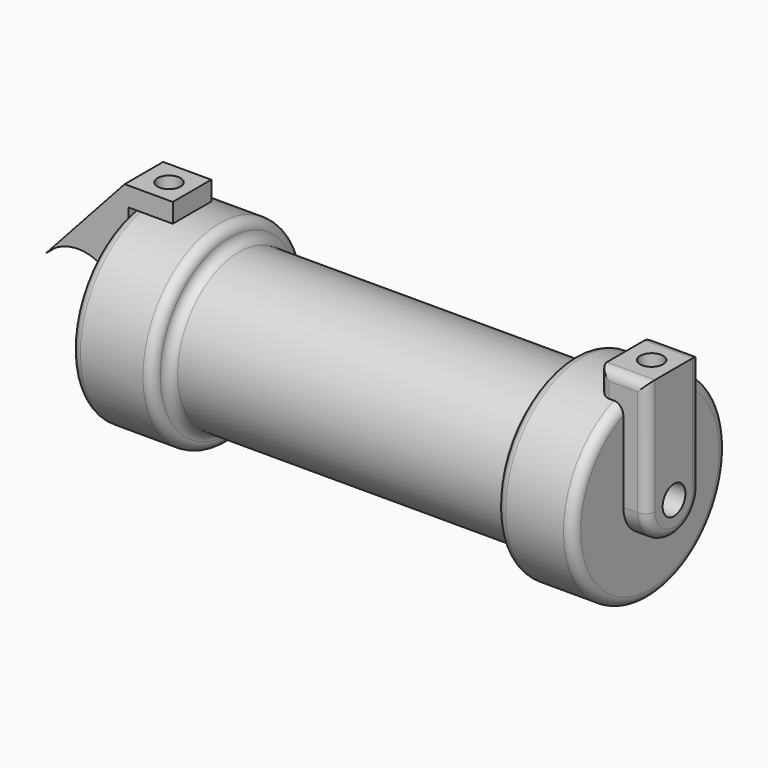
from build123d import *

# Parameters (mm, degrees)
F0_W     = 5.842
F0_H     = 12.7
F2_DEPTH = 3.175
F3_DEPTH = 0.635
F5_D     = 3.048
F5_DEPTH = 17.78
F5_TIP   = 0.9157115834
F6_R     = 1.8819905546
F7_DEPTH = 3.175
F9_D     = 3.048
F9_DEPTH = 10.414
F9_TIP   = 0.9157115834
F10_R    = 1.27
F11_R    = 1.26999


# Not quite as in the source:
# - two fillets or chamfers of one size are made in one step
# - a fillet or chamfer is up to 0.001 mm smaller than in the source, because OpenCascade refuses the exact size
# - a feature of the source that left no trace in its solid (it failed there, or was rolled back) is left out


with BuildPart() as f1:
    # F0 (on Front) → F1 (revolve)
    with BuildSketch(Plane.XZ):
        Polygon((5.842, 12.7), (5.842, 0), (66.294, 0), (66.294, 12.7), (56.134, 12.7), (56.134, 10.16), (10.16, 10.16), (10.16, 12.7), align=None)
        with Locations((2.921, 6.35)):
            Rectangle(F0_W, F0_H)
    revolve(axis=Axis((33.147, 0, 0), (-1, 0, 0)))

    # F3 (add, symmetric): a face of the model
    f3_faces = [f1.faces().sort_by_distance(p)[0] for p in [
        (10.16, 0, -10.5192102448),
    ]]
    extrude(f3_faces, amount=F3_DEPTH, both=True)

    # F6 (on face) → F7 (join, symmetric)
    with BuildSketch(Plane.YZ.offset(66.294)):
        with BuildLine():
            Line((-4.4024969223, 15.2352917939), (-4.4024969223, 11.9125153032))
            ThreePointArc((-4.4024969223, 11.9125153032), (-0.0272881349, 12.6999706833), (4.3512642127, 11.9313243084))
            Line((4.3512642127, 11.9313243084), (4.3512642127, 15.2352917939))
            Line((4.3512642127, 15.2352917939), (-0.0256163548, 15.2352917939))
            Line((-0.0256163548, 15.2352917939), (-4.4024969223, 15.2352917939))
        make_face()
        with BuildLine():
            Line((-4.4024969223, 11.9125153032), (-4.4024969223, 0.0887250123))
            ThreePointArc((-4.4024969223, 0.0887250123), (-0.2945224047, 4.3935302243), (4.3512642127, 0.6755375863))
            Line((4.3512642127, 0.6755375863), (4.3512642127, 11.9313243084))
            ThreePointArc((4.3512642127, 11.9313243084), (-0.0272881349, 12.6999706833), (-4.4024969223, 11.9125153032))
        make_face()
        with BuildLine():
            Line((-4.4024969223, 0.0887250123), (-4.4024969223, -0.0887250123))
            ThreePointArc((-4.4024969223, -0.0887250123), (0.0443647579, -4.403167388), (4.4033908842, 0))
            ThreePointArc((4.4033908842, 0), (4.3903398756, 0.3387728665), (4.3512642127, 0.6755375863))
            ThreePointArc((4.3512642127, 0.6755375863), (-0.2945224047, 4.3935302243), (-4.4024969223, 0.0887250123))
        make_face()
        Circle(F6_R, mode=Mode.SUBTRACT)
    extrude(amount=F7_DEPTH, both=True)

    # F9
    with Locations(Plane.XY.offset(15.2352917939)):
        with Locations((66.4298757911, 0.1105455449)):
            Hole(F9_D / 2, depth=F9_DEPTH)
            with Locations((0, 0, -(F9_DEPTH + F9_TIP / 2))):  # 118° drill point
                Cone(0, F9_D / 2, F9_TIP, mode=Mode.SUBTRACT)

    # F10
    f10_edges = [f1.edges().sort_by_distance(p)[0] for p in [
        (56.134, 0, -12.7),
    ]]
    fillet(f10_edges, radius=F10_R)

    # F11 (radius 1.27 in the source; OpenCascade refuses exactly that, so slightly less here)
    f11_edges = [f1.edges().sort_by_distance(p)[0] for p in [
        (10.795, 0, -12.7),
        (66.294, -4.402497, 15.235292),
        (63.119, -4.402497, 13.573904),
        (33.4645, 0, 10.16),
        (10.795, 0, -10.16),
        (56.134, 0, -10.16),
        (69.469, -4.402497, 7.573283),
        (66.294, 0.027288, -12.699971),
        (63.119, 4.351264, 13.583308),
        (69.469, 4.351264, 7.955415),
        (66.294, 4.351264, 15.235292),
        (69.469, 0.382989, -4.386704),
        (0, 0, -12.7),
    ]]
    fillet(f11_edges, radius=F11_R)


with BuildPart() as f2:
    # F0 (on Front) → F2 (new body, symmetric)
    with BuildSketch(Plane.XZ):
        with BuildLine():
            Line((-0.9398, 0), (0, 0))
            Line((0, 0), (0, 12.7))
            Line((0, 12.7), (5.842, 12.7))
            Line((5.842, 12.7), (5.842, 15.24))
            Line((5.842, 15.24), (-0.508, 15.24))
            Line((-0.508, 15.24), (-10.8806298187, 3.8475430269))
            ThreePointArc((-10.8806298187, 3.8475430269), (-4.5919612295, 5.3297205562), (-0.9398, 0))
        make_face()
    extrude(amount=F2_DEPTH, both=True)

    # F5
    with Locations(Plane.XY.offset(15.24)):
        with Locations((2.8063759673, 0)):
            Hole(F5_D / 2, depth=F5_DEPTH)
            with Locations((0, 0, -(F5_DEPTH + F5_TIP / 2))):  # 118° drill point
                Cone(0, F5_D / 2, F5_TIP, mode=Mode.SUBTRACT)


solid = Compound([f1.part, f2.part])
